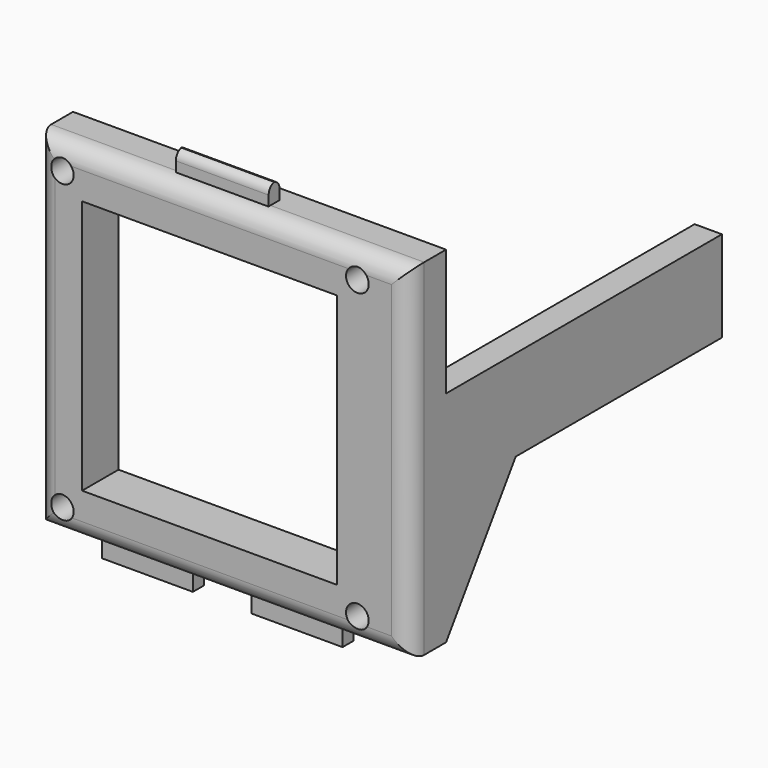
from build123d import *

# Parameters (mm, degrees)
F0_W          = 38
F0_H          = 38
F0_W_2        = 28
F0_H_2        = 28
F1_DEPTH      = 5
F2_W          = 10.2
F2_H          = 1.5
F3_DEPTH      = 2.1
F4_T1_DEPTH   = 15.2
F5_W          = 10
F5_H          = 1.5
F6_DEPTH      = 2
F8_D          = 2.5
F9_DEPTH      = 3
F10_W         = 3
F10_H         = 10
F11_DEPTH     = 37.9
F13_DEPTH     = 3
F14_T1_DEPTH  = 48
F14_T6_DEPTH  = 51
F14_T11_DEPTH = 51
F14_T16_DEPTH = 51
F14_T21_DEPTH = 51
F14_T26_DEPTH = 51
F14_T31_DEPTH = 51
F14_T37_DEPTH = 51


# Not quite as in the source:
# - a fillet or chamfer that OpenCascade refuses, or shapes differently, is made with other operations: its cross-section is extruded or revolved along the edge and cut away or added


with BuildPart() as f1:
    # F0 (on Front) → F1 (new body)
    with BuildSketch(Plane.XZ):
        Rectangle(F0_W, F0_H)
        Rectangle(F0_W_2, F0_H_2, mode=Mode.SUBTRACT)
    extrude(amount=F1_DEPTH)

    # F2 (on face) → F3 (join)
    with BuildSketch(Plane.XY.offset(19)):
        with Locations((0, -2.5)):
            Rectangle(F2_W, F2_H)
    extrude(amount=F3_DEPTH)

    # F4: fillet of radius 1 on 2 edges, made by hand

    # F4_s2 → F4_t1 (cut)
    with BuildSketch(Plane.YZ.offset(-7.6)):
        with BuildLine():
            ThreePointArc((-3.25, 20.1), (-2.9571067812, 20.8071067812), (-2.25, 21.1))
            Line((-2.25, 21.1), (-3.25, 21.1))
            Line((-3.25, 21.1), (-3.25, 20.1))
        make_face()
        with BuildLine():
            ThreePointArc((-1.75, 20.1), (-2.0428932188, 20.8071067812), (-2.75, 21.1))
            Line((-2.75, 21.1), (-1.75, 21.1))
            Line((-1.75, 21.1), (-1.75, 20.1))
        make_face()
    extrude(amount=F4_T1_DEPTH, mode=Mode.SUBTRACT)

    # F5 (on face) → F6 (join)
    with BuildSketch(Plane(origin=(0, 0, -19), x_dir=(1, 0, 0), z_dir=(0, 0, -1))):
        with Locations((-8.225, 2.5)):
            Rectangle(F5_W, F5_H)
        with Locations((8.225, 2.5)):
            Rectangle(F5_W, F5_H)
    extrude(amount=F6_DEPTH)

    # F8 (through all)
    with Locations(Plane.XZ.offset(5)):
        with Locations((16.2525195628, 16.2191219109), (-16.1783080548, 16.2191219109), (-16.1783080548, -16.3340959698), (16.2525195628, -16.3340959698)):
            Hole(F8_D / 2)

    # F9 (add): a face of the model
    f9_faces = [f1.faces().sort_by_distance(p)[0] for p in [
        (19, -2.5, 0),
    ]]
    extrude(f9_faces, amount=F9_DEPTH)

    # F10 (on face) → F11 (join)
    with BuildSketch(Plane(origin=(0, 0, 0), x_dir=(-1, 0, 0), z_dir=(0, 1, 0))):
        with Locations((-20.5, 0.0792577478)):
            Rectangle(F10_W, F10_H)
    extrude(amount=F11_DEPTH)

    # F12 (on face) → F13 (join, through all)
    with BuildSketch(Plane.YZ.offset(22)):
        Polygon((0, -4.9207422522), (0, -19), (9.5675168559, -4.9207422522), align=None)
    extrude(amount=-F13_DEPTH)

    # F14: fillet of radius 2 on 4 edges, made by hand

    # F14_s2 → F14_t1 (cut)
    with BuildSketch(Plane.XY.offset(-24)):
        with BuildLine():
            ThreePointArc((22, -3), (21.4142135624, -4.4142135624), (20, -5))
            Line((20, -5), (22, -5))
            Line((22, -5), (22, -3))
        make_face()
        with BuildLine():
            ThreePointArc((-17, -5), (-18.4142135624, -4.4142135624), (-19, -3))
            Line((-19, -3), (-19, -5))
            Line((-19, -5), (-17, -5))
        make_face()
    extrude(amount=F14_T1_DEPTH, mode=Mode.SUBTRACT)


with BuildPart() as f14_tool4:
    # F14_s5 → F14_t6 (new body)
    with BuildSketch(Plane.YZ.offset(27)):
        with BuildLine():
            ThreePointArc((-3, 19), (-4.4142135624, 18.4142135624), (-5, 17))
            Line((-5, 17), (-5, 19))
            Line((-5, 19), (-3, 19))
        make_face()
    extrude(amount=-F14_T6_DEPTH)

    split(bisect_by=Plane.YZ.offset(5.1), keep=Keep.TOP)


with BuildPart() as f1_1:
    add(f1.part)

    # F14_t3: cut F14_tool4
    add(f14_tool4.part, mode=Mode.SUBTRACT)


with BuildPart() as f14_tool9:
    # F14_s10 → F14_t11 (new body)
    with BuildSketch(Plane.YZ.offset(27)):
        with BuildLine():
            ThreePointArc((-3, 19), (-4.4142135624, 18.4142135624), (-5, 17))
            Line((-5, 17), (-5, 19))
            Line((-5, 19), (-3, 19))
        make_face()
    extrude(amount=-F14_T11_DEPTH)

    split(bisect_by=Plane.XZ.offset(3.25), keep=Keep.TOP)


with BuildPart() as f1_2:
    add(f1_1.part)

    # F14_t8: cut F14_tool9
    add(f14_tool9.part, mode=Mode.SUBTRACT)


with BuildPart() as f14_tool14:
    # F14_s15 → F14_t16 (new body)
    with BuildSketch(Plane.YZ.offset(27)):
        with BuildLine():
            ThreePointArc((-3, 19), (-4.4142135624, 18.4142135624), (-5, 17))
            Line((-5, 17), (-5, 19))
            Line((-5, 19), (-3, 19))
        make_face()
    extrude(amount=-F14_T16_DEPTH)

    split(bisect_by=Plane.YZ.offset(-5.1), keep=Keep.BOTTOM)


with BuildPart() as f1_3:
    add(f1_2.part)

    # F14_t13: cut F14_tool14
    add(f14_tool14.part, mode=Mode.SUBTRACT)


with BuildPart() as f14_tool19:
    # F14_s20 → F14_t21 (new body)
    with BuildSketch(Plane.YZ.offset(27)):
        with BuildLine():
            ThreePointArc((-3, -19), (-4.4142135624, -18.4142135624), (-5, -17))
            Line((-5, -17), (-5, -19))
            Line((-5, -19), (-3, -19))
        make_face()
    extrude(amount=-F14_T21_DEPTH)

    split(bisect_by=Plane.YZ.offset(13.225), keep=Keep.TOP)


with BuildPart() as f1_4:
    add(f1_3.part)

    # F14_t18: cut F14_tool19
    add(f14_tool19.part, mode=Mode.SUBTRACT)


with BuildPart() as f14_tool24:
    # F14_s25 → F14_t26 (new body)
    with BuildSketch(Plane.YZ.offset(27)):
        with BuildLine():
            ThreePointArc((-3, -19), (-4.4142135624, -18.4142135624), (-5, -17))
            Line((-5, -17), (-5, -19))
            Line((-5, -19), (-3, -19))
        make_face()
    extrude(amount=-F14_T26_DEPTH)

    split(bisect_by=Plane.XZ.offset(3.25), keep=Keep.TOP)


with BuildPart() as f1_5:
    add(f1_4.part)

    # F14_t23: cut F14_tool24
    add(f14_tool24.part, mode=Mode.SUBTRACT)


with BuildPart() as f14_tool29:
    # F14_s30 → F14_t31 (new body)
    with BuildSketch(Plane.YZ.offset(27)):
        with BuildLine():
            ThreePointArc((-3, -19), (-4.4142135624, -18.4142135624), (-5, -17))
            Line((-5, -17), (-5, -19))
            Line((-5, -19), (-3, -19))
        make_face()
    extrude(amount=-F14_T31_DEPTH)

    split(bisect_by=Plane.YZ.offset(3.225), keep=Keep.BOTTOM)

    split(bisect_by=Plane.YZ.offset(-3.225), keep=Keep.TOP)


with BuildPart() as f1_6:
    add(f1_5.part)

    # F14_t28: cut F14_tool29
    add(f14_tool29.part, mode=Mode.SUBTRACT)


with BuildPart() as f14_tool35:
    # F14_s36 → F14_t37 (new body)
    with BuildSketch(Plane.YZ.offset(27)):
        with BuildLine():
            ThreePointArc((-3, -19), (-4.4142135624, -18.4142135624), (-5, -17))
            Line((-5, -17), (-5, -19))
            Line((-5, -19), (-3, -19))
        make_face()
    extrude(amount=-F14_T37_DEPTH)

    split(bisect_by=Plane.YZ.offset(-13.225), keep=Keep.BOTTOM)


with BuildPart() as f1_7:
    add(f1_6.part)

    # F14_t34: cut F14_tool35
    add(f14_tool35.part, mode=Mode.SUBTRACT)


solid = f1_7.part
